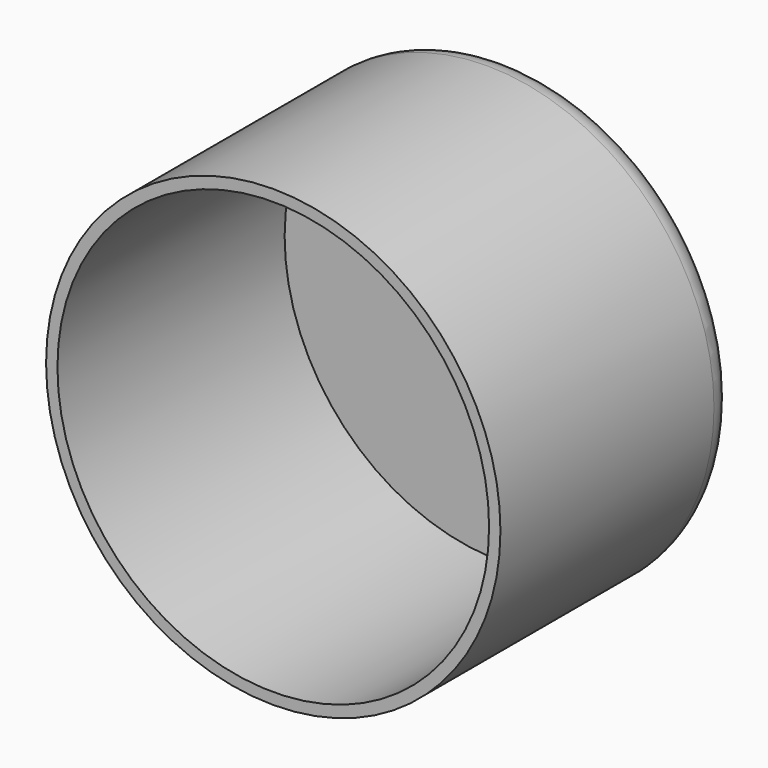
from build123d import *

# Parameters (mm, degrees)
F0_R     = 38
F1_DEPTH = 50
F2_T     = 2
F3_R     = 12.5
F4_DEPTH = 52.001
F5_R     = 5


with BuildPart() as f1:
    # F0 (on Front) → F1 (new body)
    with BuildSketch(Plane.XZ):
        Circle(F0_R)
    extrude(amount=F1_DEPTH)

    # F2
    f2_openings = [f1.faces().sort_by_distance(p)[0] for p in [
        (0, -50, 0),
    ]]
    offset(amount=F2_T, openings=f2_openings, kind=Kind.INTERSECTION)

    # F3 (on face) → F4 (cut, through all)
    with BuildSketch(Plane(origin=(0, 2, 0), x_dir=(-1, 0, 0), z_dir=(0, 1, 0))):
        Circle(F3_R)
    extrude(amount=-F4_DEPTH, mode=Mode.SUBTRACT)

    # F5
    f5_edges = [f1.edges().sort_by_distance(p)[0] for p in [
        (-40, 2, 0),
    ]]
    fillet(f5_edges, radius=F5_R)


solid = f1.part
